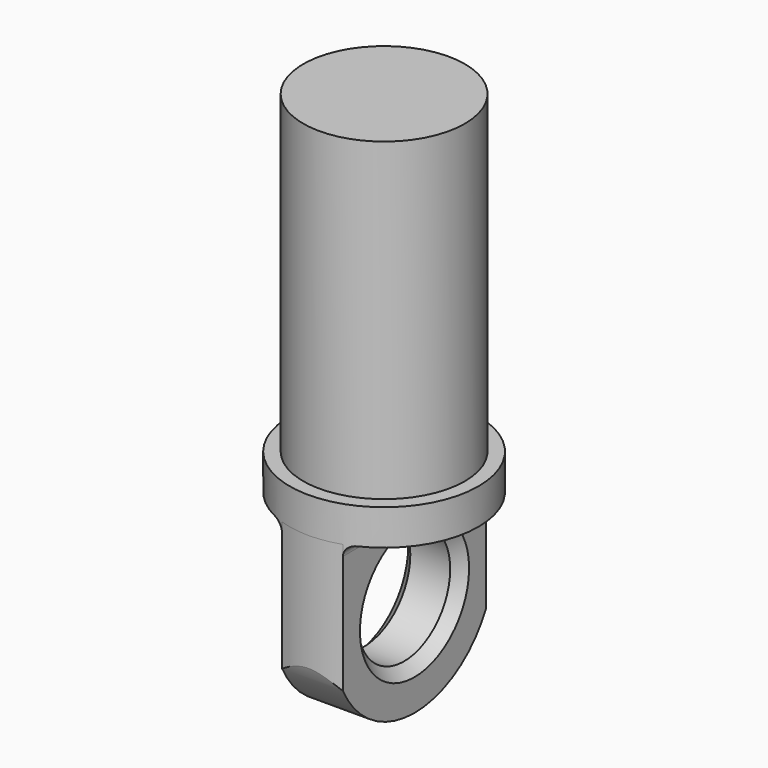
from build123d import *

# Parameters (mm, degrees)
F0_R          = 4.8895
F1_DEPTH      = 19.05
F2_R          = 5.715
F3_DEPTH      = 2.159
F4_R          = 3.4925
F5_DEPTH      = 1.8415
F5_DEPTH_BACK = 1.8415
F6_R          = 8.89
F7_DEPTH      = 25.4
F8_T4_DEPTH   = 13.9953701878
F8_S5_R       = 5.715
F8_T6_DEPTH   = 9
F8_T10_DEPTH  = 13.9953701878
F8_S11_R      = 5.715
F8_T12_DEPTH  = 9
F9_SIZE       = 0.635


# Not quite as in the source:
# - a fillet or chamfer that OpenCascade refuses, or shapes differently, is made with other operations: its cross-section is extruded or revolved along the edge and cut away or added
# - after a boolean that leaves OpenCascade's solid faulty, fix() repairs it


with BuildPart() as f1:
    # F0 (on Top) → F1 (new body)
    with BuildSketch(Plane.XY):
        Circle(F0_R)
    extrude(amount=F1_DEPTH)

    # F2 (on face) → F3 (join)
    with BuildSketch(Plane(origin=(0, 0, 0), x_dir=(1, 0, 0), z_dir=(0, 0, -1))):
        Circle(F2_R)
    extrude(amount=F3_DEPTH)

    # F4 (on Right) → F5 (join, two sides)
    with BuildSketch(Plane.YZ) as f5_sk:
        with BuildLine():
            Line((5.715, -2.159), (-5.715, -2.159))
            Line((-5.715, -2.159), (-5.715, -9.2337771034))
            ThreePointArc((-5.715, -9.2337771034), (0, -13.335), (5.715, -9.2337771034))
            Line((5.715, -9.2337771034), (5.715, -2.159))
        make_face()
        with Locations((0, -7.3025)):
            Circle(F4_R, mode=Mode.SUBTRACT)
    extrude(amount=F5_DEPTH)
    extrude(f5_sk.sketch, amount=-F5_DEPTH_BACK)

    # F6 (on face) → F7 (cut)
    with BuildSketch(Plane(origin=(0, 0, -2.159), x_dir=(1, 0, 0), z_dir=(0, 0, -1))):
        Circle(F6_R)
        with BuildLine():
            ThreePointArc((-1.8415, 5.4101850939), (3.3269394719, 4.6467944596), (5.715, 0))
            ThreePointArc((5.715, 0), (3.3269394719, -4.6467944596), (-1.8415, -5.4101850939))
            ThreePointArc((-1.8415, -5.4101850939), (-5.715, 0), (-1.8415, 5.4101850939))
        make_face(mode=Mode.SUBTRACT)
    extrude(amount=F7_DEPTH, mode=Mode.SUBTRACT)

    add(f1.part.fix(), mode=Mode.REPLACE)

    # F8: fillet of radius 0.635 on 2 edges, made by hand


with BuildPart() as f8_tool2:
    # F8_s3 → F8_t4 (new body)
    with BuildSketch(Plane.XZ.offset(-6.9976850939)):
        with BuildLine():
            ThreePointArc((2.4765, -2.159), (2.0274871939, -2.3449871939), (1.8415, -2.794))
            Line((1.8415, -2.794), (1.8415, -2.159))
            Line((1.8415, -2.159), (2.4765, -2.159))
        make_face()
    extrude(amount=F8_T4_DEPTH)

    # F8_s5 → F8_t6 (intersect, symmetric)
    with BuildSketch(Plane.XY.offset(-2.5)):
        Circle(F8_S5_R)
    extrude(amount=F8_T6_DEPTH, both=True, mode=Mode.INTERSECT)


with BuildPart() as f1_1:
    add(f1.part)

    # F8_t1: union F8_tool2
    add(f8_tool2.part)


with BuildPart() as f8_tool8:
    # F8_s9 → F8_t10 (new body)
    with BuildSketch(Plane.XZ.offset(-6.9976850939)):
        with BuildLine():
            ThreePointArc((-2.4765, -2.159), (-2.0274871939, -2.3449871939), (-1.8415, -2.794))
            Line((-1.8415, -2.794), (-1.8415, -2.159))
            Line((-1.8415, -2.159), (-2.4765, -2.159))
        make_face()
    extrude(amount=F8_T10_DEPTH)

    # F8_s11 → F8_t12 (intersect, symmetric)
    with BuildSketch(Plane.XY.offset(-2.5)):
        Circle(F8_S11_R)
    extrude(amount=F8_T12_DEPTH, both=True, mode=Mode.INTERSECT)


with BuildPart() as f1_2:
    add(f1_1.part)

    # F8_t7: union F8_tool8
    add(f8_tool8.part)

    # F9
    f9_edges = [f1_2.edges().sort_by_distance(p)[0] for p in [
        (-1.8415, -3.4925, -7.3025),
        (1.8415, -3.4925, -7.3025),
    ]]
    chamfer(f9_edges, length=F9_SIZE)


solid = f1_2.part
